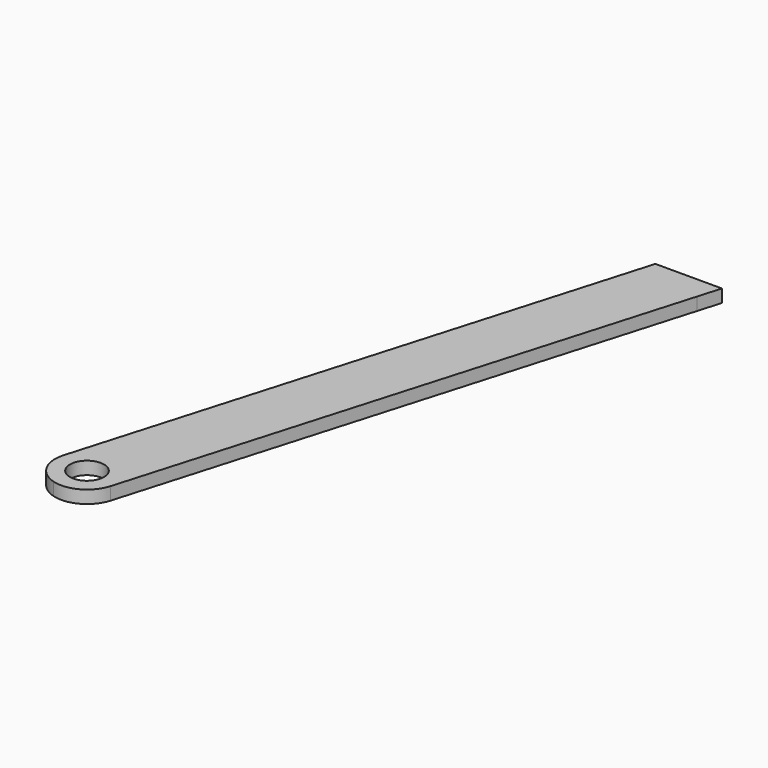
from build123d import *

# Parameters (mm, degrees)
F0_R     = 4
F1_DEPTH = 3


# Not quite as in the source:
# - a feature names something its author has since deleted; it is built from what else it names


with BuildPart() as f1:
    # F0 (on Top) → F1 (new body)
    with BuildSketch(Plane.XY):
        with BuildLine():
            Line((-11.4797556719, -12.5), (-47.2819722649, -134.6362324887))
            ThreePointArc((-47.2819722649, -134.6362324887), (-46.6657765426, -140.3433149262), (-42.1945436765, -143.9431154447))
            ThreePointArc((-42.1945436765, -143.9431154447), (-36.487461239, -143.3269197224), (-32.8876607204, -138.8556868563))
            Line((-32.8876607204, -138.8556868563), (4.0370171151, -12.8902728162))
            Line((4.0370171151, -12.8902728162), (5.6170864437, -7.5))
            Line((5.6170864437, -7.5), (-10.0140883648, -7.5))
            Line((-10.0140883648, -7.5), (-11.4797556719, -12.5))
        make_face()
        with Locations((-40.0848164926, -136.7459596725)):
            Circle(F0_R, mode=Mode.SUBTRACT)
    extrude(amount=F1_DEPTH)


solid = f1.part
